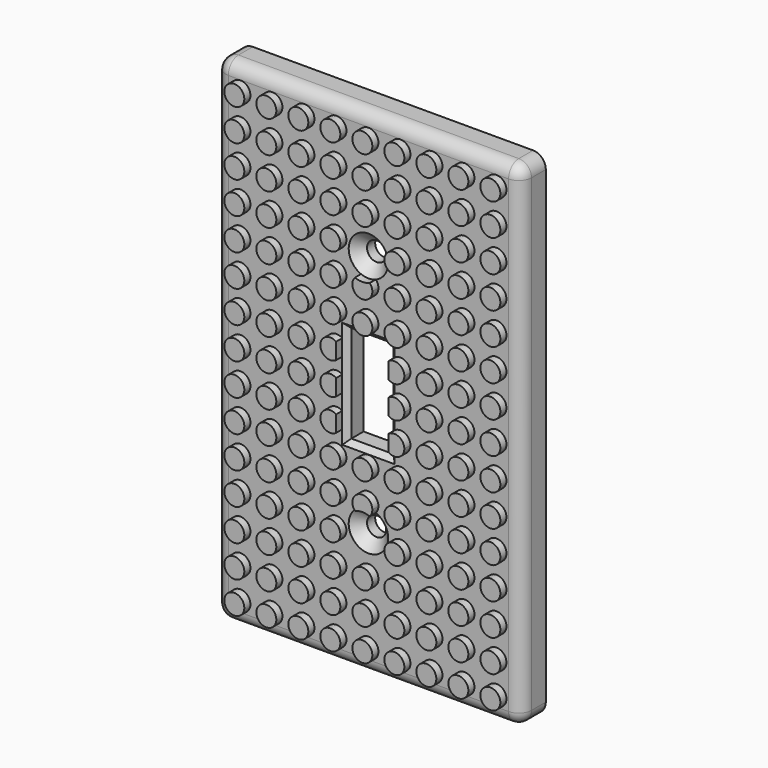
from build123d import *

# Parameters (mm, degrees)
F0_W         = 76.2
F0_H         = 123.19
F0_R         = 2.38125
F0_W_2       = 10.541
F0_H_2       = 24.257
F1_DEPTH     = 7.62
F2_SIZE      = 2.54
F3_SIZE      = 1.27
F4_T         = 2.54
F4_T3_DEPTH  = 7.2797045256
F4_T5_DEPTH  = 7.2797045256
F4_T7_DEPTH  = 7.2797045256
F4_T9_DEPTH  = 7.2797045256
F4_T11_DEPTH = 11.43
F5_W         = 57.15
F5_H         = 76.2
F5_R         = 5.9733524484
F5_W_2       = 15.621
F5_H_2       = 29.337
F6_DEPTH     = 2.54
F7_R         = 3.175
F8_R         = 3.175
F9_R         = 2.4892
F10_DEPTH    = 1.905


# Not quite as in the source:
# - a shell that OpenCascade refuses in one call is made with other operations: the cavity is built on its own and cut out
# - a feature names something its author has since deleted; it is built from what else it names


with BuildPart() as f1:
    # F0 (on Front) → F1 (new body)
    with BuildSketch(Plane.XZ):
        Rectangle(F0_W, F0_H)
        with Locations((0, -30.1625)):
            Circle(F0_R, mode=Mode.SUBTRACT)
        Rectangle(F0_W_2, F0_H_2, mode=Mode.SUBTRACT)
        with Locations((0, 30.1625)):
            Circle(F0_R, mode=Mode.SUBTRACT)
    extrude(amount=F1_DEPTH)

    # F2
    f2_edges = [f1.edges().sort_by_distance(p)[0] for p in [
        (-2.38125, -7.62, 30.1625),
        (-2.38125, -7.62, -30.1625),
    ]]
    chamfer(f2_edges, length=F2_SIZE)

    # F3
    f3_edges = [f1.edges().sort_by_distance(p)[0] for p in [
        (0, -7.62, -12.1285),
        (0, -7.62, 12.1285),
        (5.2705, -7.62, 0),
        (-5.2705, -7.62, 0),
    ]]
    chamfer(f3_edges, length=F3_SIZE)

    # F4: shell of thickness 2.54, made by hand


with BuildPart() as f4_core1:
    # F4_t2: copy of F1
    add(f1.part)

    # the walls: a layer under each face that stays
    f4_faces = [f4_core1.faces().sort_by_distance(p)[0] for p in [
        (-25.4, -7.62, -41.0633333333),
        (0, -6.985, -12.7635),
        (5.9055, -6.985, 0),
        (-5.9055, -6.985, 0),
        (0, -6.985, 12.7635),
        (-3.65125, -6.35, 30.1625),
        (-38.1, -3.81, 0),
        (0, -3.81, -61.595),
        (38.1, -3.81, 0),
        (0, -3.81, 61.595),
        (-3.65125, -6.35, -30.1625),
        (0, -3.175, -12.1285),
        (5.2705, -3.175, 0),
        (-5.2705, -3.175, 0),
        (0, -3.175, 12.1285),
        (-2.38125, -2.54, 30.1625),
        (-2.38125, -2.54, -30.1625),
    ]]
    thicken(f4_faces, amount=-F4_T, mode=Mode.SUBTRACT)

    # F4_s4 → F4_t3 (cut)
    with BuildSketch(Plane(origin=(10.6528030171, -10.6528030171, -10.6528030171), x_dir=(-0.7071067812, -0.7071067812, 0), z_dir=(-0.5773502692, 0.5773502692, 0.5773502692))):
        Polygon((0.8014217703, -5.1368324772), (-0.5066782297, -7.3585340481), (-1.7766782297, -6.6252992062), (-1.7766782297, -5.1588295224), align=None)
    extrude(amount=F4_T3_DEPTH, mode=Mode.SUBTRACT)

    # F4_s6 → F4_t5 (cut)
    with BuildSketch(Plane(origin=(-10.6528030171, -10.6528030171, -10.6528030171), x_dir=(-0.7071067812, 0.7071067812, 0), z_dir=(0.5773502692, 0.5773502692, 0.5773502692))):
        Polygon((-0.8014217703, -5.1368324772), (0.5066782297, -7.3585340481), (1.7766782297, -6.6252992062), (1.7766782297, -5.1588295224), align=None)
    extrude(amount=F4_T5_DEPTH, mode=Mode.SUBTRACT)

    # F4_s8 → F4_t7 (cut)
    with BuildSketch(Plane(origin=(10.6528030171, -10.6528030171, 10.6528030171), x_dir=(-0.7071067812, -0.7071067812, 0), z_dir=(-0.5773502692, 0.5773502692, -0.5773502692))):
        Polygon((0.8014217703, 5.1368324772), (-1.7766782297, 5.1588295224), (-1.7766782297, 6.6252992062), (-0.5066782297, 7.3585340481), align=None)
    extrude(amount=F4_T7_DEPTH, mode=Mode.SUBTRACT)

    # F4_s10 → F4_t9 (cut)
    with BuildSketch(Plane(origin=(-10.6528030171, -10.6528030171, 10.6528030171), x_dir=(-0.7071067812, 0.7071067812, 0), z_dir=(0.5773502692, 0.5773502692, -0.5773502692))):
        Polygon((-0.8014217703, 5.1368324772), (1.7766782297, 5.1588295224), (1.7766782297, 6.6252992062), (0.5066782297, 7.3585340481), align=None)
    extrude(amount=F4_T9_DEPTH, mode=Mode.SUBTRACT)

    # F4_s12 → F4_t11 (cut)
    with BuildSketch(Plane.XZ.offset(-2.54)):
        Polygon((5.2451, -12.1031), (5.2705, -14.6685), (7.8105, -14.6685), (7.8105, -12.1285), align=None)
        Polygon((-5.2451, -12.1031), (-5.2705, -14.6685), (-7.8105, -14.6685), (-7.8105, -12.1285), align=None)
        Polygon((5.2451, 12.1031), (7.8105, 12.1285), (7.8105, 14.6685), (5.2705, 14.6685), align=None)
        Polygon((-5.2451, 12.1031), (-7.8105, 12.1285), (-7.8105, 14.6685), (-5.2705, 14.6685), align=None)
    extrude(amount=F4_T11_DEPTH, mode=Mode.SUBTRACT)


with BuildPart() as f1_1:
    add(f1.part)

    # what is left inside the walls is the cavity
    f4_cavity = [f4_core1.part.solids().sort_by_distance(p)[0] for p in [
        (0, -0.0254, -19.685),
    ]]
    add(f4_cavity, mode=Mode.SUBTRACT)

    # F5 (on face) → F6 (cut)
    with BuildSketch(Plane(origin=(0, 0, 0), x_dir=(-1, 0, 0), z_dir=(0, 1, 0))):
        Rectangle(F5_W, F5_H)
        with Locations((0, -30.1625)):
            Circle(F5_R, mode=Mode.SUBTRACT)
        Rectangle(F5_W_2, F5_H_2, mode=Mode.SUBTRACT)
        with Locations((0, 30.1625)):
            Circle(F5_R, mode=Mode.SUBTRACT)
        with Locations((0, -30.1625)):
            Circle(F5_R)
        Rectangle(F5_W_2, F5_H_2)
        with Locations((0, 30.1625)):
            Circle(F5_R)
    extrude(amount=-F6_DEPTH, mode=Mode.SUBTRACT)

    # F7
    f7_edges = [f1_1.edges().sort_by_distance(p)[0] for p in [
        (38.1, -3.81, 61.595),
        (38.1, -3.81, -61.595),
        (-38.1, -3.81, -61.595),
        (-38.1, -3.81, 61.595),
    ]]
    fillet(f7_edges, radius=F7_R)

    # F8
    f8_edges = [f1_1.edges().sort_by_distance(p)[0] for p in [
        (0, -7.62, 61.595),
        (-38.1, -7.62, 0),
        (-37.170064, -7.62, 60.665064),
        (-37.170064, -7.62, -60.665064),
        (0, -7.62, -61.595),
        (37.170064, -7.62, 60.665064),
        (37.170064, -7.62, -60.665064),
        (38.1, -7.62, 0),
    ]]
    fillet(f8_edges, radius=F8_R)

    # F9 (on face) → F10 (join)
    with BuildSketch(Plane.XZ.offset(7.62)):
        with Locations((0, 15.9512)):
            Circle(F9_R)
        with BuildLine():
            ThreePointArc((-1.8433850061, 25.5995367872), (-0.8965385331, 21.6046597591), (2.4892, 23.9268))
            ThreePointArc((2.4892, 23.9268), (2.3221402409, 24.8233385331), (1.8433850061, 25.5995367872))
            ThreePointArc((1.8433850061, 25.5995367872), (0, 25.24125), (-1.8433850061, 25.5995367872))
        make_face()
        with Locations((0, 39.878)):
            Circle(F9_R)
        with Locations((0, 47.8536)):
            Circle(F9_R)
        with Locations((0, 55.8292)):
            Circle(F9_R)
        with BuildLine():
            ThreePointArc((6.5405, -2.0338644571), (9.1209963768, -2.2100189547), (10.4648, 0))
            ThreePointArc((10.4648, 0), (9.1209963768, 2.2100189547), (6.5405, 2.0338644571))
            Line((6.5405, 2.0338644571), (6.5405, -2.0338644571))
        make_face()
        with BuildLine():
            Line((6.5405, 10.0094644571), (6.5405, 5.9417355429))
            ThreePointArc((6.5405, 5.9417355429), (9.1209963768, 5.7655810453), (10.4648, 7.9756))
            ThreePointArc((10.4648, 7.9756), (9.1209963768, 10.1856189547), (6.5405, 10.0094644571))
        make_face()
        with BuildLine():
            ThreePointArc((10.4648, -7.9756), (9.1209963768, -5.7655810453), (6.5405, -5.9417355429))
            Line((6.5405, -5.9417355429), (6.5405, -10.0094644571))
            ThreePointArc((6.5405, -10.0094644571), (9.1209963768, -10.1856189547), (10.4648, -7.9756))
        make_face()
        with BuildLine():
            Line((-6.5405, 5.9417355429), (-6.5405, 10.0094644571))
            ThreePointArc((-6.5405, 10.0094644571), (-10.4648, 7.9756), (-6.5405, 5.9417355429))
        make_face()
        with BuildLine():
            ThreePointArc((-6.5405, -5.9417355429), (-10.4648, -7.9756), (-6.5405, -10.0094644571))
            Line((-6.5405, -10.0094644571), (-6.5405, -5.9417355429))
        make_face()
        with BuildLine():
            Line((-6.5405, -2.0338644571), (-6.5405, 2.0338644571))
            ThreePointArc((-6.5405, 2.0338644571), (-10.4648, 0), (-6.5405, -2.0338644571))
        make_face()
        with Locations((7.9756, 15.9512)):
            Circle(F9_R)
        with Locations((7.9756, 23.9268)):
            Circle(F9_R)
        with Locations((7.9756, 31.9024)):
            Circle(F9_R)
        with Locations((7.9756, 39.878)):
            Circle(F9_R)
        with Locations((7.9756, 47.8536)):
            Circle(F9_R)
        with Locations((7.9756, 55.8292)):
            Circle(F9_R)
        with Locations((15.9512, 0)):
            Circle(F9_R)
        with Locations((15.9512, 7.9756)):
            Circle(F9_R)
        with Locations((15.9512, 15.9512)):
            Circle(F9_R)
        with Locations((15.9512, 23.9268)):
            Circle(F9_R)
        with Locations((15.9512, 31.9024)):
            Circle(F9_R)
        with Locations((15.9512, 39.878)):
            Circle(F9_R)
        with Locations((15.9512, 47.8536)):
            Circle(F9_R)
        with Locations((15.9512, 55.8292)):
            Circle(F9_R)
        with Locations((23.9268, 0)):
            Circle(F9_R)
        with Locations((23.9268, 7.9756)):
            Circle(F9_R)
        with Locations((23.9268, 15.9512)):
            Circle(F9_R)
        with Locations((23.9268, 23.9268)):
            Circle(F9_R)
        with Locations((23.9268, 31.9024)):
            Circle(F9_R)
        with Locations((23.9268, 39.878)):
            Circle(F9_R)
        with Locations((23.9268, 47.8536)):
            Circle(F9_R)
        with Locations((23.9268, 55.8292)):
            Circle(F9_R)
        with Locations((31.9024, 0)):
            Circle(F9_R)
        with Locations((31.9024, 7.9756)):
            Circle(F9_R)
        with Locations((31.9024, 15.9512)):
            Circle(F9_R)
        with Locations((31.9024, 23.9268)):
            Circle(F9_R)
        with Locations((31.9024, 31.9024)):
            Circle(F9_R)
        with Locations((31.9024, 39.878)):
            Circle(F9_R)
        with Locations((31.9024, 47.8536)):
            Circle(F9_R)
        with Locations((31.9024, 55.8292)):
            Circle(F9_R)
        with Locations((-15.9512, 0)):
            Circle(F9_R)
        with Locations((-23.9268, 0)):
            Circle(F9_R)
        with Locations((-31.9024, 0)):
            Circle(F9_R)
        with Locations((-15.9512, -7.9756)):
            Circle(F9_R)
        with Locations((-23.9268, -7.9756)):
            Circle(F9_R)
        with Locations((-31.9024, -7.9756)):
            Circle(F9_R)
        with Locations((0, -15.9512)):
            Circle(F9_R)
        with Locations((-7.9756, -15.9512)):
            Circle(F9_R)
        with Locations((-15.9512, -15.9512)):
            Circle(F9_R)
        with Locations((-23.9268, -15.9512)):
            Circle(F9_R)
        with Locations((-31.9024, -15.9512)):
            Circle(F9_R)
        with BuildLine():
            ThreePointArc((1.8433850061, -25.5995367872), (2.3221402409, -24.8233385331), (2.4892, -23.9268))
            ThreePointArc((2.4892, -23.9268), (-0.8965385331, -21.6046597591), (-1.8433850061, -25.5995367872))
            ThreePointArc((-1.8433850061, -25.5995367872), (0, -25.24125), (1.8433850061, -25.5995367872))
        make_face()
        with Locations((-7.9756, -23.9268)):
            Circle(F9_R)
        with Locations((-15.9512, -23.9268)):
            Circle(F9_R)
        with Locations((-23.9268, -23.9268)):
            Circle(F9_R)
        with Locations((-31.9024, -23.9268)):
            Circle(F9_R)
        with Locations((-7.9756, -31.9024)):
            Circle(F9_R)
        with Locations((-15.9512, -31.9024)):
            Circle(F9_R)
        with Locations((-23.9268, -31.9024)):
            Circle(F9_R)
        with Locations((-31.9024, -31.9024)):
            Circle(F9_R)
        with Locations((0, -39.878)):
            Circle(F9_R)
        with Locations((-7.9756, -39.878)):
            Circle(F9_R)
        with Locations((-15.9512, -39.878)):
            Circle(F9_R)
        with Locations((-23.9268, -39.878)):
            Circle(F9_R)
        with Locations((-31.9024, -39.878)):
            Circle(F9_R)
        with Locations((0, -47.8536)):
            Circle(F9_R)
        with Locations((-7.9756, -47.8536)):
            Circle(F9_R)
        with Locations((-15.9512, -47.8536)):
            Circle(F9_R)
        with Locations((-23.9268, -47.8536)):
            Circle(F9_R)
        with Locations((-31.9024, -47.8536)):
            Circle(F9_R)
        with Locations((0, -55.8292)):
            Circle(F9_R)
        with Locations((-7.9756, -55.8292)):
            Circle(F9_R)
        with Locations((-15.9512, -55.8292)):
            Circle(F9_R)
        with Locations((-23.9268, -55.8292)):
            Circle(F9_R)
        with Locations((-31.9024, -55.8292)):
            Circle(F9_R)
        with Locations((-7.9756, 15.9512)):
            Circle(F9_R)
        with Locations((-7.9756, 23.9268)):
            Circle(F9_R)
        with Locations((-7.9756, 31.9024)):
            Circle(F9_R)
        with Locations((-7.9756, 39.878)):
            Circle(F9_R)
        with Locations((-7.9756, 47.8536)):
            Circle(F9_R)
        with Locations((-7.9756, 55.8292)):
            Circle(F9_R)
        with Locations((-15.9512, 7.9756)):
            Circle(F9_R)
        with Locations((-15.9512, 15.9512)):
            Circle(F9_R)
        with Locations((-15.9512, 23.9268)):
            Circle(F9_R)
        with Locations((-15.9512, 31.9024)):
            Circle(F9_R)
        with Locations((-15.9512, 39.878)):
            Circle(F9_R)
        with Locations((-15.9512, 47.8536)):
            Circle(F9_R)
        with Locations((-15.9512, 55.8292)):
            Circle(F9_R)
        with Locations((-23.9268, 7.9756)):
            Circle(F9_R)
        with Locations((-23.9268, 15.9512)):
            Circle(F9_R)
        with Locations((-23.9268, 23.9268)):
            Circle(F9_R)
        with Locations((-23.9268, 31.9024)):
            Circle(F9_R)
        with Locations((-23.9268, 39.878)):
            Circle(F9_R)
        with Locations((-23.9268, 47.8536)):
            Circle(F9_R)
        with Locations((-23.9268, 55.8292)):
            Circle(F9_R)
        with Locations((-31.9024, 7.9756)):
            Circle(F9_R)
        with Locations((-31.9024, 15.9512)):
            Circle(F9_R)
        with Locations((-31.9024, 23.9268)):
            Circle(F9_R)
        with Locations((-31.9024, 31.9024)):
            Circle(F9_R)
        with Locations((-31.9024, 39.878)):
            Circle(F9_R)
        with Locations((-31.9024, 47.8536)):
            Circle(F9_R)
        with Locations((-31.9024, 55.8292)):
            Circle(F9_R)
        with Locations((7.9756, -15.9512)):
            Circle(F9_R)
        with Locations((7.9756, -23.9268)):
            Circle(F9_R)
        with Locations((7.9756, -31.9024)):
            Circle(F9_R)
        with Locations((7.9756, -39.878)):
            Circle(F9_R)
        with Locations((7.9756, -47.8536)):
            Circle(F9_R)
        with Locations((7.9756, -55.8292)):
            Circle(F9_R)
        with Locations((15.9512, -7.9756)):
            Circle(F9_R)
        with Locations((15.9512, -15.9512)):
            Circle(F9_R)
        with Locations((15.9512, -23.9268)):
            Circle(F9_R)
        with Locations((15.9512, -31.9024)):
            Circle(F9_R)
        with Locations((15.9512, -39.878)):
            Circle(F9_R)
        with Locations((15.9512, -47.8536)):
            Circle(F9_R)
        with Locations((15.9512, -55.8292)):
            Circle(F9_R)
        with Locations((23.9268, -7.9756)):
            Circle(F9_R)
        with Locations((23.9268, -15.9512)):
            Circle(F9_R)
        with Locations((23.9268, -23.9268)):
            Circle(F9_R)
        with Locations((23.9268, -31.9024)):
            Circle(F9_R)
        with Locations((23.9268, -39.878)):
            Circle(F9_R)
        with Locations((23.9268, -47.8536)):
            Circle(F9_R)
        with Locations((23.9268, -55.8292)):
            Circle(F9_R)
        with Locations((31.9024, -7.9756)):
            Circle(F9_R)
        with Locations((31.9024, -15.9512)):
            Circle(F9_R)
        with Locations((31.9024, -23.9268)):
            Circle(F9_R)
        with Locations((31.9024, -31.9024)):
            Circle(F9_R)
        with Locations((31.9024, -39.878)):
            Circle(F9_R)
        with Locations((31.9024, -47.8536)):
            Circle(F9_R)
        with Locations((31.9024, -55.8292)):
            Circle(F9_R)
    extrude(amount=F10_DEPTH)


solid = f1_1.part
